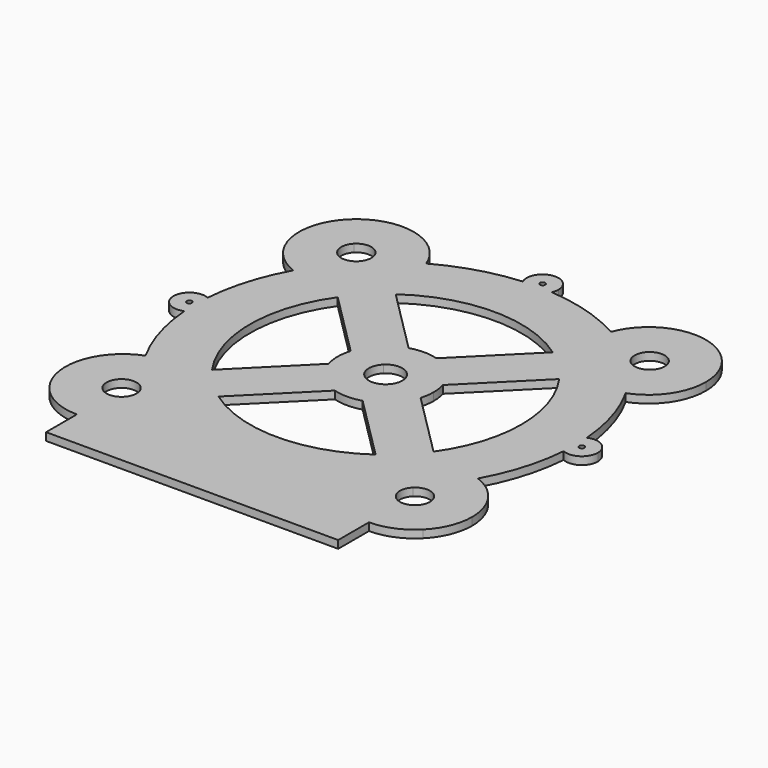
from build123d import *

# Parameters (mm, degrees)
F0_R     = 1.5875
F1_DEPTH = 4.7625


# Not quite as in the source:
# - a length typed as a fraction of an inch, garbled in the dataset ("3 / 203.2 mm" for 3/8 in), is restored


with BuildPart() as f1:
    # F0 (on Top) → F1 (new body)
    with BuildSketch(Plane.XY):
        with BuildLine():
            ThreePointArc((-101.9853941355, 56.6876837116), (-93.1446500572, 70.2750899486), (-82.5061031123, 82.5061031123))
            Line((-82.5061031123, 82.5061031123), (-83.5163819259, 83.5163819259))
            ThreePointArc((-83.5163819259, 83.5163819259), (-96.5377533015, 83.5163819259), (-96.5377533015, 96.5377533015))
            Line((-96.5377533015, 96.5377533015), (-114.4982655436, 114.4982655436))
            ThreePointArc((-114.4982655436, 114.4982655436), (-124.0057759655, 82.180930941), (-101.9853941355, 56.6876837116))
        make_face()
        with BuildLine():
            ThreePointArc((-82.5061031123, 82.5061031123), (-70.2750899486, 93.1446500572), (-56.6876837116, 101.9853941355))
            ThreePointArc((-56.6876837116, 101.9853941355), (-82.180930941, 124.0057759655), (-114.4982655436, 114.4982655436))
            Line((-114.4982655436, 114.4982655436), (-96.5377533015, 96.5377533015))
            ThreePointArc((-96.5377533015, 96.5377533015), (-86.5035099102, 98.5336884093), (-80.8195676137, 90.0270676137))
            ThreePointArc((-80.8195676137, 90.0270676137), (-81.5204468181, 86.5035099102), (-83.5163819259, 83.5163819259))
            Line((-83.5163819259, 83.5163819259), (-82.5061031123, 82.5061031123))
        make_face()
        with BuildLine():
            ThreePointArc((-54.4439560883, 89.6229560883), (-55.0094328066, 95.9051568993), (-56.6876837116, 101.9853941355))
            ThreePointArc((-56.6876837116, 101.9853941355), (-70.2750899486, 93.1446500572), (-82.5061031123, 82.5061031123))
            Line((-82.5061031123, 82.5061031123), (-64.7476466329, 64.7476466329))
            ThreePointArc((-64.7476466329, 64.7476466329), (-57.1217980141, 76.1605356211), (-54.4439560883, 89.6229560883))
        make_face()
        with BuildLine():
            Line((-64.7476466329, 64.7476466329), (-82.5061031123, 82.5061031123))
            ThreePointArc((-82.5061031123, 82.5061031123), (-93.1446500572, 70.2750899486), (-101.9853941355, 56.6876837116))
            ThreePointArc((-101.9853941355, 56.6876837116), (-82.180930941, 55.2401362111), (-64.7476466329, 64.7476466329))
        make_face()
        with BuildLine():
            ThreePointArc((-67.954647167, 48.1980837006), (-63.6582986892, 53.7448634941), (-58.9104801542, 58.9104801542))
            Line((-58.9104801542, 58.9104801542), (-64.7476466329, 64.7476466329))
            ThreePointArc((-64.7476466329, 64.7476466329), (-82.180930941, 55.2401362111), (-101.9853941355, 56.6876837116))
            ThreePointArc((-101.9853941355, 56.6876837116), (-111.7478973152, 33.5696521758), (-116.3414153151, 8.8988304868))
            ThreePointArc((-116.3414153151, 8.8988304868), (-112.1716877299, 5.2905130832), (-110.617, 0))
            ThreePointArc((-110.617, 0), (-112.1716877299, -5.2905130832), (-116.3414153151, -8.8988304868))
            ThreePointArc((-116.3414153151, -8.8988304868), (-111.7478973152, -33.5696521758), (-101.9853941355, -56.6876837116))
            ThreePointArc((-101.9853941355, -56.6876837116), (-82.180930941, -55.2401362111), (-64.7476466329, -64.7476466329))
            Line((-64.7476466329, -64.7476466329), (-58.9104801542, -58.9104801542))
            ThreePointArc((-58.9104801542, -58.9104801542), (-63.6582986892, -53.7448634941), (-67.954647167, -48.1980837006))
            ThreePointArc((-67.954647167, -48.1980837006), (-83.312, 0), (-67.954647167, 48.1980837006))
        make_face()
        with BuildLine():
            Line((58.9104801542, 58.9104801542), (64.7476466329, 64.7476466329))
            ThreePointArc((64.7476466329, 64.7476466329), (55.2401362111, 82.180930941), (56.6876837116, 101.9853941355))
            ThreePointArc((56.6876837116, 101.9853941355), (33.5696521758, 111.7478973152), (8.8988304868, 116.3414153151))
            ThreePointArc((8.8988304868, 116.3414153151), (0, 110.617), (-8.8988304868, 116.3414153151))
            ThreePointArc((-8.8988304868, 116.3414153151), (-33.5696521758, 111.7478973152), (-56.6876837116, 101.9853941355))
            ThreePointArc((-56.6876837116, 101.9853941355), (-55.0094328066, 95.9051568993), (-54.4439560883, 89.6229560883))
            ThreePointArc((-54.4439560883, 89.6229560883), (-57.1217980141, 76.1605356211), (-64.7476466329, 64.7476466329))
            Line((-64.7476466329, 64.7476466329), (-58.9104801542, 58.9104801542))
            ThreePointArc((-58.9104801542, 58.9104801542), (-53.7448634941, 63.6582986892), (-48.1980837006, 67.954647167))
            ThreePointArc((-48.1980837006, 67.954647167), (0, 83.312), (48.1980837006, 67.954647167))
            ThreePointArc((48.1980837006, 67.954647167), (53.7448634941, 63.6582986892), (58.9104801542, 58.9104801542))
        make_face()
        with BuildLine():
            ThreePointArc((116.3414153151, -8.8988304868), (110.617, 0), (116.3414153151, 8.8988304868))
            ThreePointArc((116.3414153151, 8.8988304868), (111.7478973152, 33.5696521758), (101.9853941355, 56.6876837116))
            ThreePointArc((101.9853941355, 56.6876837116), (82.180930941, 55.2401362111), (64.7476466329, 64.7476466329))
            Line((64.7476466329, 64.7476466329), (58.9104801542, 58.9104801542))
            ThreePointArc((58.9104801542, 58.9104801542), (63.6582986892, 53.7448634941), (67.954647167, 48.1980837006))
            ThreePointArc((67.954647167, 48.1980837006), (79.3798680673, 25.2928031189), (83.312, 0))
            ThreePointArc((83.312, 0), (79.3798680673, -25.2928031189), (67.954647167, -48.1980837006))
            ThreePointArc((67.954647167, -48.1980837006), (63.6582986892, -53.7448634941), (58.9104801542, -58.9104801542))
            Line((58.9104801542, -58.9104801542), (64.7476466329, -64.7476466329))
            ThreePointArc((64.7476466329, -64.7476466329), (82.180930941, -55.2401362111), (101.9853941355, -56.6876837116))
            ThreePointArc((101.9853941355, -56.6876837116), (111.7478973152, -33.5696521758), (116.3414153151, -8.8988304868))
        make_face()
        with BuildLine():
            ThreePointArc((56.6876837116, -101.9853941355), (55.2401362111, -82.180930941), (64.7476466329, -64.7476466329))
            Line((64.7476466329, -64.7476466329), (58.9104801542, -58.9104801542))
            ThreePointArc((58.9104801542, -58.9104801542), (53.7448634941, -63.6582986892), (48.1980837006, -67.954647167))
            ThreePointArc((48.1980837006, -67.954647167), (0, -83.312), (-48.1980837006, -67.954647167))
            ThreePointArc((-48.1980837006, -67.954647167), (-53.7448634941, -63.6582986892), (-58.9104801542, -58.9104801542))
            Line((-58.9104801542, -58.9104801542), (-64.7476466329, -64.7476466329))
            ThreePointArc((-64.7476466329, -64.7476466329), (-57.1217980141, -76.1605356211), (-54.4439560883, -89.6229560883))
            ThreePointArc((-54.4439560883, -89.6229560883), (-55.0094328066, -95.9051568993), (-56.6876837116, -101.9853941355))
            ThreePointArc((-56.6876837116, -101.9853941355), (0, -116.68125), (56.6876837116, -101.9853941355))
        make_face()
        with BuildLine():
            ThreePointArc((-82.5061031123, -82.5061031123), (-70.2750899486, -93.1446500572), (-56.6876837116, -101.9853941355))
            ThreePointArc((-56.6876837116, -101.9853941355), (-55.0094328066, -95.9051568993), (-54.4439560883, -89.6229560883))
            ThreePointArc((-54.4439560883, -89.6229560883), (-57.1217980141, -76.1605356211), (-64.7476466329, -64.7476466329))
            Line((-64.7476466329, -64.7476466329), (-82.5061031123, -82.5061031123))
        make_face()
        with BuildLine():
            ThreePointArc((-101.9853941355, -56.6876837116), (-93.1446500572, -70.2750899486), (-82.5061031123, -82.5061031123))
            Line((-82.5061031123, -82.5061031123), (-64.7476466329, -64.7476466329))
            ThreePointArc((-64.7476466329, -64.7476466329), (-82.180930941, -55.2401362111), (-101.9853941355, -56.6876837116))
        make_face()
        with BuildLine():
            ThreePointArc((56.6876837116, -101.9853941355), (70.2750899486, -93.1446500572), (82.5061031123, -82.5061031123))
            Line((82.5061031123, -82.5061031123), (64.7476466329, -64.7476466329))
            ThreePointArc((64.7476466329, -64.7476466329), (55.2401362111, -82.180930941), (56.6876837116, -101.9853941355))
        make_face()
        with BuildLine():
            ThreePointArc((82.5061031123, -82.5061031123), (93.1446500572, -70.2750899486), (101.9853941355, -56.6876837116))
            ThreePointArc((101.9853941355, -56.6876837116), (82.180930941, -55.2401362111), (64.7476466329, -64.7476466329))
            Line((64.7476466329, -64.7476466329), (82.5061031123, -82.5061031123))
        make_face()
        with BuildLine():
            ThreePointArc((64.7476466329, 64.7476466329), (82.180930941, 55.2401362111), (101.9853941355, 56.6876837116))
            ThreePointArc((101.9853941355, 56.6876837116), (93.1446500572, 70.2750899486), (82.5061031123, 82.5061031123))
            Line((82.5061031123, 82.5061031123), (64.7476466329, 64.7476466329))
        make_face()
        with BuildLine():
            Line((64.7476466329, 64.7476466329), (82.5061031123, 82.5061031123))
            ThreePointArc((82.5061031123, 82.5061031123), (70.2750899486, 93.1446500572), (56.6876837116, 101.9853941355))
            ThreePointArc((56.6876837116, 101.9853941355), (55.2401362111, 82.180930941), (64.7476466329, 64.7476466329))
        make_face()
        with BuildLine():
            ThreePointArc((82.5061031123, 82.5061031123), (93.1446500572, 70.2750899486), (101.9853941355, 56.6876837116))
            ThreePointArc((101.9853941355, 56.6876837116), (118.5405999157, 69.5896858493), (124.8019560883, 89.6229560883))
            ThreePointArc((124.8019560883, 89.6229560883), (122.1241141625, 103.0853765554), (114.4982655436, 114.4982655436))
            Line((114.4982655436, 114.4982655436), (96.5377533015, 96.5377533015))
            ThreePointArc((96.5377533015, 96.5377533015), (98.5336884093, 93.5506253172), (99.2345676137, 90.0270676137))
            ThreePointArc((99.2345676137, 90.0270676137), (93.5506253172, 81.5204468181), (83.5163819259, 83.5163819259))
            Line((83.5163819259, 83.5163819259), (82.5061031123, 82.5061031123))
        make_face()
        with BuildLine():
            ThreePointArc((56.6876837116, 101.9853941355), (70.2750899486, 93.1446500572), (82.5061031123, 82.5061031123))
            Line((82.5061031123, 82.5061031123), (83.5163819259, 83.5163819259))
            ThreePointArc((83.5163819259, 83.5163819259), (83.5163819259, 96.5377533015), (96.5377533015, 96.5377533015))
            Line((96.5377533015, 96.5377533015), (114.4982655436, 114.4982655436))
            ThreePointArc((114.4982655436, 114.4982655436), (82.180930941, 124.0057759655), (56.6876837116, 101.9853941355))
        make_face()
        with BuildLine():
            Line((-83.5163819259, -83.5163819259), (-82.5061031123, -82.5061031123))
            ThreePointArc((-82.5061031123, -82.5061031123), (-93.1446500572, -70.2750899486), (-101.9853941355, -56.6876837116))
            ThreePointArc((-101.9853941355, -56.6876837116), (-124.0057759655, -82.180930941), (-114.4982655436, -114.4982655436))
            Line((-114.4982655436, -114.4982655436), (-96.5377533015, -96.5377533015))
            ThreePointArc((-96.5377533015, -96.5377533015), (-96.5377533015, -83.5163819259), (-83.5163819259, -83.5163819259))
        make_face()
        with BuildLine():
            ThreePointArc((-89.6229560883, -124.8019560883), (-69.5896858493, -118.5405999157), (-56.6876837116, -101.9853941355))
            ThreePointArc((-56.6876837116, -101.9853941355), (-70.2750899486, -93.1446500572), (-82.5061031123, -82.5061031123))
            Line((-82.5061031123, -82.5061031123), (-83.5163819259, -83.5163819259))
            ThreePointArc((-83.5163819259, -83.5163819259), (-81.5204468181, -86.5035099102), (-80.8195676137, -90.0270676137))
            ThreePointArc((-80.8195676137, -90.0270676137), (-86.5035099102, -98.5336884093), (-96.5377533015, -96.5377533015))
            Line((-96.5377533015, -96.5377533015), (-114.4982655436, -114.4982655436))
            ThreePointArc((-114.4982655436, -114.4982655436), (-103.0853765554, -122.1241141625), (-89.6229560883, -124.8019560883))
        make_face()
        with BuildLine():
            Line((83.5163819259, -83.5163819259), (82.5061031123, -82.5061031123))
            ThreePointArc((82.5061031123, -82.5061031123), (70.2750899486, -93.1446500572), (56.6876837116, -101.9853941355))
            ThreePointArc((56.6876837116, -101.9853941355), (69.5896858493, -118.5405999157), (89.6229560883, -124.8019560883))
            ThreePointArc((89.6229560883, -124.8019560883), (103.0853765554, -122.1241141625), (114.4982655436, -114.4982655436))
            Line((114.4982655436, -114.4982655436), (96.5377533015, -96.5377533015))
            ThreePointArc((96.5377533015, -96.5377533015), (83.5163819259, -96.5377533015), (83.5163819259, -83.5163819259))
        make_face()
        with BuildLine():
            ThreePointArc((124.8019560883, -89.6229560883), (118.5405999157, -69.5896858493), (101.9853941355, -56.6876837116))
            ThreePointArc((101.9853941355, -56.6876837116), (93.1446500572, -70.2750899486), (82.5061031123, -82.5061031123))
            Line((82.5061031123, -82.5061031123), (83.5163819259, -83.5163819259))
            ThreePointArc((83.5163819259, -83.5163819259), (93.5506253172, -81.5204468181), (99.2345676137, -90.0270676137))
            ThreePointArc((99.2345676137, -90.0270676137), (98.5336884093, -93.5506253172), (96.5377533015, -96.5377533015))
            Line((96.5377533015, -96.5377533015), (114.4982655436, -114.4982655436))
            ThreePointArc((114.4982655436, -114.4982655436), (122.1241141625, -103.0853765554), (124.8019560883, -89.6229560883))
        make_face()
        with BuildLine():
            ThreePointArc((116.3414153151, 8.8988304868), (116.5962603759, 4.4526585218), (116.68125, 0))
            ThreePointArc((116.68125, 0), (116.5962603759, -4.4526585218), (116.3414153151, -8.8988304868))
            ThreePointArc((116.3414153151, -8.8988304868), (125.6865130832, -8.2243122701), (130.175, 0))
            ThreePointArc((130.175, 0), (125.6865130832, 8.2243122701), (116.3414153151, 8.8988304868))
        make_face()
        with Locations((120.396, 0)):
            Circle(F0_R, mode=Mode.SUBTRACT)
        with BuildLine():
            ThreePointArc((116.3414153151, -8.8988304868), (116.5962603759, -4.4526585218), (116.68125, 0))
            ThreePointArc((116.68125, 0), (116.5962603759, 4.4526585218), (116.3414153151, 8.8988304868))
            ThreePointArc((116.3414153151, 8.8988304868), (110.617, 0), (116.3414153151, -8.8988304868))
        make_face()
        with BuildLine():
            ThreePointArc((-116.3414153151, 8.8988304868), (-116.68125, 0), (-116.3414153151, -8.8988304868))
            ThreePointArc((-116.3414153151, -8.8988304868), (-112.1716877299, -5.2905130832), (-110.617, 0))
            ThreePointArc((-110.617, 0), (-112.1716877299, 5.2905130832), (-116.3414153151, 8.8988304868))
        make_face()
        with BuildLine():
            ThreePointArc((-116.3414153151, 8.8988304868), (-130.175, 0), (-116.3414153151, -8.8988304868))
            ThreePointArc((-116.3414153151, -8.8988304868), (-116.68125, 0), (-116.3414153151, 8.8988304868))
        make_face()
        with Locations((-120.396, 0)):
            Circle(F0_R, mode=Mode.SUBTRACT)
        with BuildLine():
            ThreePointArc((-8.8988304868, 116.3414153151), (0, 110.617), (8.8988304868, 116.3414153151))
            ThreePointArc((8.8988304868, 116.3414153151), (0, 116.68125), (-8.8988304868, 116.3414153151))
        make_face()
        with BuildLine():
            ThreePointArc((-8.8988304868, 116.3414153151), (0, 116.68125), (8.8988304868, 116.3414153151))
            ThreePointArc((8.8988304868, 116.3414153151), (9.5564246539, 118.3214907003), (9.779, 120.396))
            ThreePointArc((9.779, 120.396), (-2.0745092997, 129.9524246539), (-8.8988304868, 116.3414153151))
        make_face()
        with Locations((0, 120.396)):
            Circle(F0_R, mode=Mode.SUBTRACT)
        with BuildLine():
            ThreePointArc((89.6229560883, -124.8019560883), (69.5896858493, -118.5405999157), (56.6876837116, -101.9853941355))
            ThreePointArc((56.6876837116, -101.9853941355), (0, -116.68125), (-56.6876837116, -101.9853941355))
            ThreePointArc((-56.6876837116, -101.9853941355), (-69.5896858493, -118.5405999157), (-89.6229560883, -124.8019560883))
            Line((-89.6229560883, -124.8019560883), (-89.6229560883, -148.43125))
            Line((-89.6229560883, -148.43125), (89.6229560883, -148.43125))
            Line((89.6229560883, -148.43125), (89.6229560883, -124.8019560883))
        make_face()
        with BuildLine():
            ThreePointArc((48.1980837006, -67.954647167), (53.7448634941, -63.6582986892), (58.9104801542, -58.9104801542))
            Line((58.9104801542, -58.9104801542), (20.8790954815, -20.8790954815))
            ThreePointArc((20.8790954815, -20.8790954815), (15.1554294108, -25.3413933245), (8.5161787951, -28.2727422614))
            Line((8.5161787951, -28.2727422614), (48.1980837006, -67.954647167))
        make_face()
        with BuildLine():
            Line((20.8790954815, -20.8790954815), (58.9104801542, -58.9104801542))
            ThreePointArc((58.9104801542, -58.9104801542), (63.6582986892, -53.7448634941), (67.954647167, -48.1980837006))
            Line((67.954647167, -48.1980837006), (28.2727422614, -8.5161787951))
            ThreePointArc((28.2727422614, -8.5161787951), (25.3413933245, -15.1554294108), (20.8790954815, -20.8790954815))
        make_face()
        with BuildLine():
            Line((9.8782817332, -9.8782817332), (20.8790954815, -20.8790954815))
            ThreePointArc((20.8790954815, -20.8790954815), (25.3413933245, -15.1554294108), (28.2727422614, -8.5161787951))
            Line((28.2727422614, -8.5161787951), (19.7565634664, 0))
            Line((19.7565634664, 0), (9.8782817332, -9.8782817332))
        make_face()
        with BuildLine():
            ThreePointArc((8.5161787951, -28.2727422614), (15.1554294108, -25.3413933245), (20.8790954815, -20.8790954815))
            Line((20.8790954815, -20.8790954815), (9.8782817332, -9.8782817332))
            Line((9.8782817332, -9.8782817332), (0, -19.7565634664))
            Line((0, -19.7565634664), (8.5161787951, -28.2727422614))
        make_face()
        with BuildLine():
            Line((-8.5161787951, -28.2727422614), (0, -19.7565634664))
            Line((0, -19.7565634664), (-9.8782817332, -9.8782817332))
            Line((-9.8782817332, -9.8782817332), (-20.8790954815, -20.8790954815))
            ThreePointArc((-20.8790954815, -20.8790954815), (-15.1554294108, -25.3413933245), (-8.5161787951, -28.2727422614))
        make_face()
        with BuildLine():
            ThreePointArc((-58.9104801542, -58.9104801542), (-53.7448634941, -63.6582986892), (-48.1980837006, -67.954647167))
            Line((-48.1980837006, -67.954647167), (-8.5161787951, -28.2727422614))
            ThreePointArc((-8.5161787951, -28.2727422614), (-15.1554294108, -25.3413933245), (-20.8790954815, -20.8790954815))
            Line((-20.8790954815, -20.8790954815), (-58.9104801542, -58.9104801542))
        make_face()
        with BuildLine():
            ThreePointArc((-67.954647167, -48.1980837006), (-63.6582986892, -53.7448634941), (-58.9104801542, -58.9104801542))
            Line((-58.9104801542, -58.9104801542), (-20.8790954815, -20.8790954815))
            ThreePointArc((-20.8790954815, -20.8790954815), (-25.3413933245, -15.1554294108), (-28.2727422614, -8.5161787951))
            Line((-28.2727422614, -8.5161787951), (-67.954647167, -48.1980837006))
        make_face()
        with BuildLine():
            ThreePointArc((-8.5161787951, -28.2727422614), (0, -29.5275), (8.5161787951, -28.2727422614))
            Line((8.5161787951, -28.2727422614), (0, -19.7565634664))
            Line((0, -19.7565634664), (-8.5161787951, -28.2727422614))
        make_face()
        with BuildLine():
            ThreePointArc((29.5275, 0), (29.2121263637, 4.3040596607), (28.2727422614, 8.5161787951))
            Line((28.2727422614, 8.5161787951), (19.7565634664, 0))
            Line((19.7565634664, 0), (28.2727422614, -8.5161787951))
            ThreePointArc((28.2727422614, -8.5161787951), (29.2121263637, -4.3040596607), (29.5275, 0))
        make_face()
        with BuildLine():
            Line((-20.8790954815, -20.8790954815), (-9.8782817332, -9.8782817332))
            Line((-9.8782817332, -9.8782817332), (-19.7565634664, 0))
            Line((-19.7565634664, 0), (-28.2727422614, -8.5161787951))
            ThreePointArc((-28.2727422614, -8.5161787951), (-25.3413933245, -15.1554294108), (-20.8790954815, -20.8790954815))
        make_face()
        with BuildLine():
            Line((-28.2727422614, -8.5161787951), (-19.7565634664, 0))
            Line((-19.7565634664, 0), (-28.2727422614, 8.5161787951))
            ThreePointArc((-28.2727422614, 8.5161787951), (-29.5275, 0), (-28.2727422614, -8.5161787951))
        make_face()
        with BuildLine():
            Line((-19.7565634664, 0), (-9.8782817332, 9.8782817332))
            Line((-9.8782817332, 9.8782817332), (-20.8790954815, 20.8790954815))
            ThreePointArc((-20.8790954815, 20.8790954815), (-25.3413933245, 15.1554294108), (-28.2727422614, 8.5161787951))
            Line((-28.2727422614, 8.5161787951), (-19.7565634664, 0))
        make_face()
        with BuildLine():
            Line((-9.8782817332, 9.8782817332), (0, 19.7565634664))
            Line((0, 19.7565634664), (-8.5161787951, 28.2727422614))
            ThreePointArc((-8.5161787951, 28.2727422614), (-15.1554294108, 25.3413933245), (-20.8790954815, 20.8790954815))
            Line((-20.8790954815, 20.8790954815), (-9.8782817332, 9.8782817332))
        make_face()
        with BuildLine():
            Line((0, 19.7565634664), (8.5161787951, 28.2727422614))
            ThreePointArc((8.5161787951, 28.2727422614), (0, 29.5275), (-8.5161787951, 28.2727422614))
            Line((-8.5161787951, 28.2727422614), (0, 19.7565634664))
        make_face()
        with BuildLine():
            Line((9.8782817332, 9.8782817332), (20.8790954815, 20.8790954815))
            ThreePointArc((20.8790954815, 20.8790954815), (15.1554294108, 25.3413933245), (8.5161787951, 28.2727422614))
            Line((8.5161787951, 28.2727422614), (0, 19.7565634664))
            Line((0, 19.7565634664), (9.8782817332, 9.8782817332))
        make_face()
        with BuildLine():
            ThreePointArc((28.2727422614, 8.5161787951), (25.3413933245, 15.1554294108), (20.8790954815, 20.8790954815))
            Line((20.8790954815, 20.8790954815), (9.8782817332, 9.8782817332))
            Line((9.8782817332, 9.8782817332), (19.7565634664, 0))
            Line((19.7565634664, 0), (28.2727422614, 8.5161787951))
        make_face()
        with BuildLine():
            Line((19.7565634664, 0), (9.8782817332, 9.8782817332))
            Line((9.8782817332, 9.8782817332), (7.2740074581, 7.2740074581))
            ThreePointArc((7.2740074581, 7.2740074581), (9.5039487509, 3.9366644687), (10.287, 0))
            ThreePointArc((10.287, 0), (9.5039487509, -3.9366644687), (7.2740074581, -7.2740074581))
            Line((7.2740074581, -7.2740074581), (9.8782817332, -9.8782817332))
            Line((9.8782817332, -9.8782817332), (19.7565634664, 0))
        make_face()
        with BuildLine():
            Line((0, -19.7565634664), (9.8782817332, -9.8782817332))
            Line((9.8782817332, -9.8782817332), (7.2740074581, -7.2740074581))
            ThreePointArc((7.2740074581, -7.2740074581), (0, -10.287), (-7.2740074581, -7.2740074581))
            Line((-7.2740074581, -7.2740074581), (-9.8782817332, -9.8782817332))
            Line((-9.8782817332, -9.8782817332), (0, -19.7565634664))
        make_face()
        with BuildLine():
            ThreePointArc((-7.2740074581, -7.2740074581), (-10.287, 0), (-7.2740074581, 7.2740074581))
            Line((-7.2740074581, 7.2740074581), (-9.8782817332, 9.8782817332))
            Line((-9.8782817332, 9.8782817332), (-19.7565634664, 0))
            Line((-19.7565634664, 0), (-9.8782817332, -9.8782817332))
            Line((-9.8782817332, -9.8782817332), (-7.2740074581, -7.2740074581))
        make_face()
        with BuildLine():
            Line((7.2740074581, 7.2740074581), (9.8782817332, 9.8782817332))
            Line((9.8782817332, 9.8782817332), (0, 19.7565634664))
            Line((0, 19.7565634664), (-9.8782817332, 9.8782817332))
            Line((-9.8782817332, 9.8782817332), (-7.2740074581, 7.2740074581))
            ThreePointArc((-7.2740074581, 7.2740074581), (0, 10.287), (7.2740074581, 7.2740074581))
        make_face()
        with BuildLine():
            ThreePointArc((67.954647167, 48.1980837006), (63.6582986892, 53.7448634941), (58.9104801542, 58.9104801542))
            Line((58.9104801542, 58.9104801542), (20.8790954815, 20.8790954815))
            ThreePointArc((20.8790954815, 20.8790954815), (25.3413933245, 15.1554294108), (28.2727422614, 8.5161787951))
            Line((28.2727422614, 8.5161787951), (67.954647167, 48.1980837006))
        make_face()
        with BuildLine():
            Line((20.8790954815, 20.8790954815), (58.9104801542, 58.9104801542))
            ThreePointArc((58.9104801542, 58.9104801542), (53.7448634941, 63.6582986892), (48.1980837006, 67.954647167))
            Line((48.1980837006, 67.954647167), (8.5161787951, 28.2727422614))
            ThreePointArc((8.5161787951, 28.2727422614), (15.1554294108, 25.3413933245), (20.8790954815, 20.8790954815))
        make_face()
        with BuildLine():
            Line((-8.5161787951, 28.2727422614), (-48.1980837006, 67.954647167))
            ThreePointArc((-48.1980837006, 67.954647167), (-53.7448634941, 63.6582986892), (-58.9104801542, 58.9104801542))
            Line((-58.9104801542, 58.9104801542), (-20.8790954815, 20.8790954815))
            ThreePointArc((-20.8790954815, 20.8790954815), (-15.1554294108, 25.3413933245), (-8.5161787951, 28.2727422614))
        make_face()
        with BuildLine():
            Line((-20.8790954815, 20.8790954815), (-58.9104801542, 58.9104801542))
            ThreePointArc((-58.9104801542, 58.9104801542), (-63.6582986892, 53.7448634941), (-67.954647167, 48.1980837006))
            Line((-67.954647167, 48.1980837006), (-28.2727422614, 8.5161787951))
            ThreePointArc((-28.2727422614, 8.5161787951), (-25.3413933245, 15.1554294108), (-20.8790954815, 20.8790954815))
        make_face()
    extrude(amount=F1_DEPTH)


solid = f1.part
